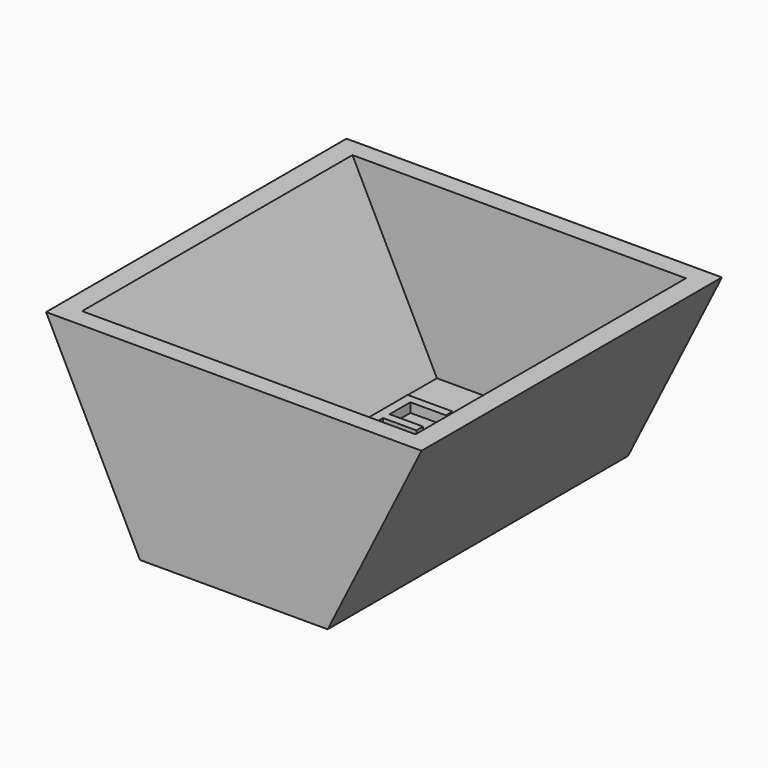
from build123d import *

# Parameters (mm, degrees)
F1_DEPTH     = 50.8
F2_T         = -2.54
F3_TEXT_SIZE = 15.2746305305
F4_DEPTH     = 1.27


# Not quite as in the source:
# - Text() gives the source's letters only with a copy of the font that has no kerning and outlines rounded to 1/6400 em; it was checked with that copy


with BuildPart() as f1:
    # F0 (on Front) → F1 (new body)
    with BuildSketch(Plane.XZ):
        Polygon((-28.8237119008, 22.8739220768), (-54.2237119008, 22.8739220768), (-41.5237119008, -2.5260779232), (-28.8237119008, -2.5260779232), align=None)
        Polygon((-3.4237119008, 22.8739220768), (-28.8237119008, 22.8739220768), (-28.8237119008, -2.5260779232), (-16.1237119008, -2.5260779232), align=None)
    extrude(amount=F1_DEPTH)

    # F2
    f2_openings = [f1.faces().sort_by_distance(p)[0] for p in [
        (-28.823712, -25.4, 22.873922),
    ]]
    offset(amount=F2_T, openings=f2_openings)

    # F3 (on face) → F4 (join)
    with BuildSketch(Plane.XY.offset(0.0139220768)):
        with Locations((-39.9539055694, -20.2594638323)):
            Text('EL', F3_TEXT_SIZE, font='Open Sans', text_align=(TextAlign.LEFT, TextAlign.BOTTOM))
        with Locations((-39.9539055694, -41.0329613537)):
            Text('OK', F3_TEXT_SIZE, font='Open Sans', text_align=(TextAlign.LEFT, TextAlign.BOTTOM))
    extrude(amount=F4_DEPTH)


solid = f1.part
